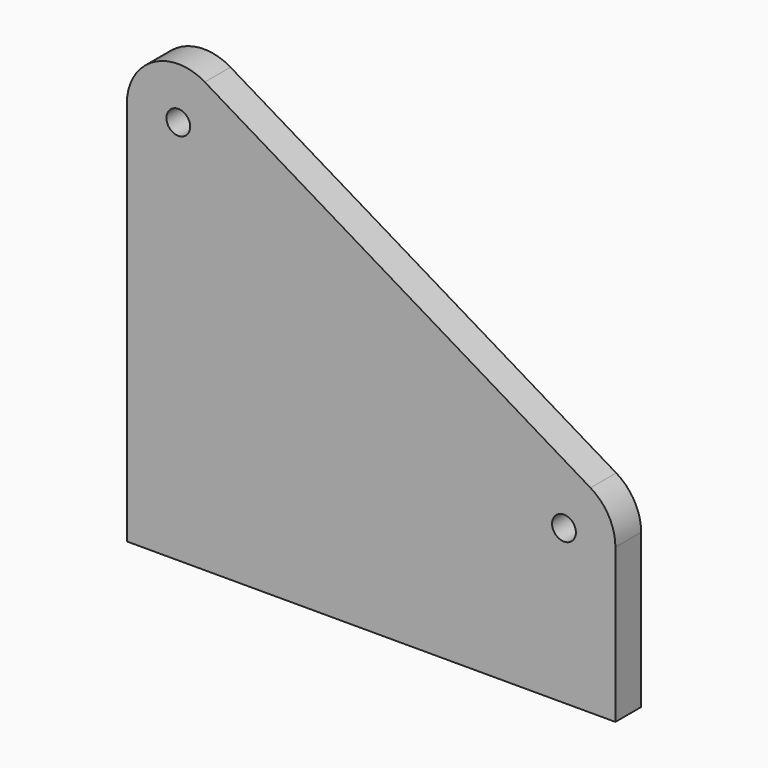
from build123d import *

# Parameters (mm, degrees)
F0_R     = 1.85
F1_DEPTH = 2.5


# Not quite as in the source:
# - a feature names something its author has since deleted; it is built from what else it names


with BuildPart() as f1:
    # F0 (on Front) → F1 (new body, symmetric)
    with BuildSketch(Plane.XZ):
        with BuildLine():
            Line((4.1206300291, 6.8571428571), (-55.8793699709, 42.9126556118))
            ThreePointArc((-55.8793699709, 42.9126556118), (-63.9392232589, 43.0184517976), (-68, 36.0555127546))
            Line((-68, 36.0555127546), (-68, -23.9444872454))
            Line((-68, -23.9444872454), (8, -23.9444872454))
            Line((8, -23.9444872454), (8, 0))
            ThreePointArc((8, 0), (6.962939043, 3.9392232589), (4.1206300291, 6.8571428571))
        make_face()
        Circle(F0_R, mode=Mode.SUBTRACT)
        with Locations((-60, 36.0555127546)):
            Circle(F0_R, mode=Mode.SUBTRACT)
    extrude(amount=F1_DEPTH, both=True)


solid = f1.part
